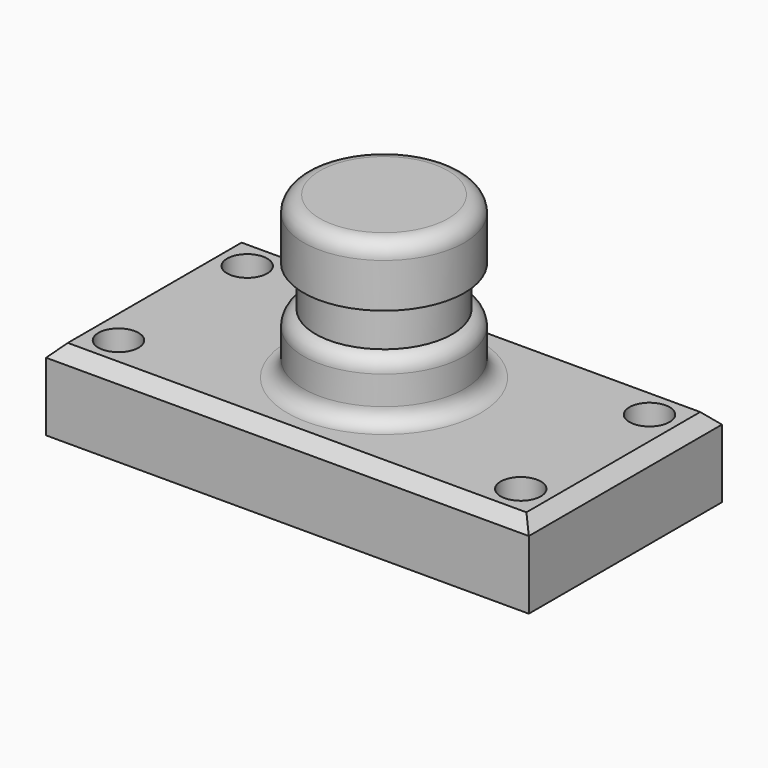
from build123d import *

# Parameters (mm, degrees)
F0_W     = 152.4
F0_H     = 76.2
F1_DEPTH = 25.4
F2_R     = 6.35
F3_DEPTH = 25.401
F4_SIZE  = 3.81


# Not quite as in the source:
# - a fillet or chamfer that OpenCascade refuses, or shapes differently, is made with other operations: its cross-section is extruded or revolved along the edge and cut away or added


with BuildPart() as f1:
    # F0 (on Top) → F1 (new body)
    with BuildSketch(Plane.XY):
        Rectangle(F0_W, F0_H)
    extrude(amount=F1_DEPTH)

    # F2 (on face) → F3 (cut, through all)
    with BuildSketch(Plane.XY.offset(25.4)):
        with Locations((-63.5, 25.4)):
            Circle(F2_R)
        with Locations((63.5, 25.4)):
            Circle(F2_R)
        with Locations((63.5, -25.4)):
            Circle(F2_R)
        with Locations((-63.5, -25.4)):
            Circle(F2_R)
    extrude(amount=-F3_DEPTH, mode=Mode.SUBTRACT)

    # F4
    f4_edges = [f1.edges().sort_by_distance(p)[0] for p in [
        (0, -38.1, 25.4),
        (-76.2, 0, 25.4),
        (0, 38.1, 25.4),
        (76.2, 0, 25.4),
    ]]
    chamfer(f4_edges, length=F4_SIZE)

    # F5 (on Front) → F6 (revolve)
    with BuildSketch(Plane.XZ):
        Polygon((0, 76.2), (0, 25.4), (25.4, 25.4), (25.4, 44.45), (21.59, 44.45), (21.59, 57.15), (25.4, 57.15), (25.4, 76.2), align=None)
    revolve(axis=Axis((0, 0, 50.8), (0, 0, 1)))

    # F7: fillet of radius 5.08 on 3 edges, made by hand

    # F7_s1 → F7_t2 (revolve)
    with BuildSketch(Plane.XZ):
        with BuildLine():
            ThreePointArc((30.48, 25.4), (26.8878975516, 26.8878975516), (25.4, 30.48))
            Line((25.4, 30.48), (25.4, 25.4))
            Line((25.4, 25.4), (30.48, 25.4))
        make_face()
    revolve(axis=Axis((0, 0, 25.4), (0, 0, 1)))

    # F7_s3 → F7_t4 (revolve, cut)
    with BuildSketch(Plane.XZ):
        with BuildLine():
            ThreePointArc((25.4, 39.5313111503), (24.3360926284, 42.6421631237), (21.59, 44.45))
            Line((21.59, 44.45), (25.4, 44.45))
            Line((25.4, 44.45), (25.4, 39.5313111503))
        make_face()
    revolve(axis=Axis((0, 0, 44.45), (0, 0, 1)), mode=Mode.SUBTRACT)

    # F7_s5 → F7_t6 (revolve, cut)
    with BuildSketch(Plane.XZ):
        with BuildLine():
            ThreePointArc((25.4, 71.12), (23.9121024484, 74.7121024484), (20.32, 76.2))
            Line((20.32, 76.2), (25.4, 76.2))
            Line((25.4, 76.2), (25.4, 71.12))
        make_face()
    revolve(axis=Axis((0, 0, 76.2), (0, 0, 1)), mode=Mode.SUBTRACT)


solid = f1.part
